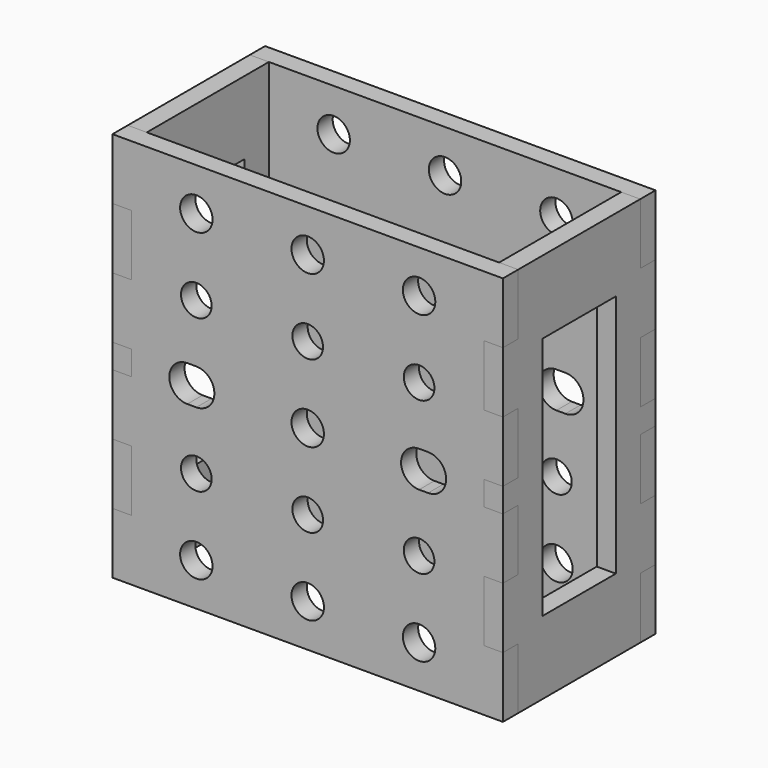
from build123d import *

# Parameters (mm, degrees)
F2_R     = 2.7
F2_R_2   = 2.55
F3_DEPTH = 3.175
F6_W     = 3.175
F6_H     = 10.16
F6_H_2   = 4.04
F6_W_2   = 15.24
F6_H_3   = 40.64
F7_DEPTH = 3.175


# Not quite as in the source:
# - a variable given as a bare number and used for a length is read in inches; the dataset says mm whatever the document's units were
# - a feature names something its author has since deleted; it is built from what else it names


with BuildPart() as f3:
    # F2 (on offset) → F3 (new body)
    with BuildSketch(Plane.XZ.offset(12.7)):
        Polygon((32.5, 22.34), (32.5, 32.5), (-32.5, 32.5), (-32.5, 22.34), (-29.325, 22.34), (-29.325, 12.18), (-32.5, 12.18), (-32.5, 2.02), (-29.325, 2.02), (-29.325, 0), (-29.325, -2.02), (-32.5, -2.02), (-32.5, -12.18), (-29.325, -12.18), (-29.325, -22.34), (-32.5, -22.34), (-32.5, -32.5), (32.5, -32.5), (32.5, -22.34), (29.325, -22.34), (29.325, -12.18), (32.5, -12.18), (32.5, -2.02), (29.325, -2.02), (29.325, 0), (29.325, 2.02), (32.5, 2.02), (32.5, 12.18), (29.325, 12.18), (29.325, 22.34), align=None)
        with Locations((-18.542, -25.4)):
            Circle(F2_R, mode=Mode.SUBTRACT)
        with Locations((-18.542, -12.7)):
            Circle(F2_R_2, mode=Mode.SUBTRACT)
        with Locations((0, -25.4)):
            Circle(F2_R, mode=Mode.SUBTRACT)
        with Locations((18.542, -25.4)):
            Circle(F2_R, mode=Mode.SUBTRACT)
        with Locations((0, -12.7)):
            Circle(F2_R_2, mode=Mode.SUBTRACT)
        with Locations((18.542, -12.7)):
            Circle(F2_R_2, mode=Mode.SUBTRACT)
        with BuildLine():
            Line((-18.542, -3), (-20.042, -3))
            ThreePointArc((-20.042, -3), (-23.042, 0), (-20.042, 3))
            Line((-20.042, 3), (-18.542, 3))
            ThreePointArc((-18.542, 3), (-15.542, 0), (-18.542, -3))
        make_face(mode=Mode.SUBTRACT)
        with Locations((-18.542, 12.7)):
            Circle(F2_R_2, mode=Mode.SUBTRACT)
        with Locations((-18.542, 25.4)):
            Circle(F2_R, mode=Mode.SUBTRACT)
        Circle(F2_R, mode=Mode.SUBTRACT)
        with Locations((0, 12.7)):
            Circle(F2_R_2, mode=Mode.SUBTRACT)
        with BuildLine():
            ThreePointArc((18.542, -3), (15.542, 0), (18.542, 3))
            Line((18.542, 3), (20.042, 3))
            ThreePointArc((20.042, 3), (23.042, 0), (20.042, -3))
            Line((20.042, -3), (18.542, -3))
        make_face(mode=Mode.SUBTRACT)
        with Locations((18.542, 12.7)):
            Circle(F2_R_2, mode=Mode.SUBTRACT)
        with Locations((0, 25.4)):
            Circle(F2_R, mode=Mode.SUBTRACT)
        with Locations((18.542, 25.4)):
            Circle(F2_R, mode=Mode.SUBTRACT)
    extrude(amount=F3_DEPTH)


with BuildPart() as f4_1:
    # F4: instance of F3
    add(f3.part.mirror(Plane.XZ))


with BuildPart() as f7:
    # F6 (on face) → F7 (new body)
    with BuildSketch(Plane(origin=(-29.325, 0, 0), x_dir=(0, -1, 0), z_dir=(-1, 0, 0))):
        with Locations((-14.2875, 17.26)):
            Rectangle(F6_W, F6_H)
        with Locations((-14.2875, 0)):
            Rectangle(F6_W, F6_H_2)
        Polygon((-12.7, 22.34), (-12.7, 12.18), (-12.7, 2.02), (-12.7, -2.02), (-12.7, -12.18), (-12.7, -22.34), (-12.7, -32.5), (12.7, -32.5), (12.7, -22.34), (12.7, -12.18), (12.7, -2.02), (12.7, 2.02), (12.7, 12.18), (12.7, 22.34), (12.7, 32.5), (-12.7, 32.5), align=None)
        Rectangle(F6_W_2, F6_H_3, mode=Mode.SUBTRACT)
        with Locations((14.2875, -17.26)):
            Rectangle(F6_W, F6_H)
        with Locations((14.2875, 0)):
            Rectangle(F6_W, F6_H_2)
        with Locations((14.2875, 17.26)):
            Rectangle(F6_W, F6_H)
        with Locations((-14.2875, -17.26)):
            Rectangle(F6_W, F6_H)
    extrude(amount=F7_DEPTH)


with BuildPart() as f8_1:
    # F8: instance of F7
    add(f7.part.mirror(Plane.YZ))


solid = Compound([f3.part, f4_1.part, f7.part, f8_1.part])
